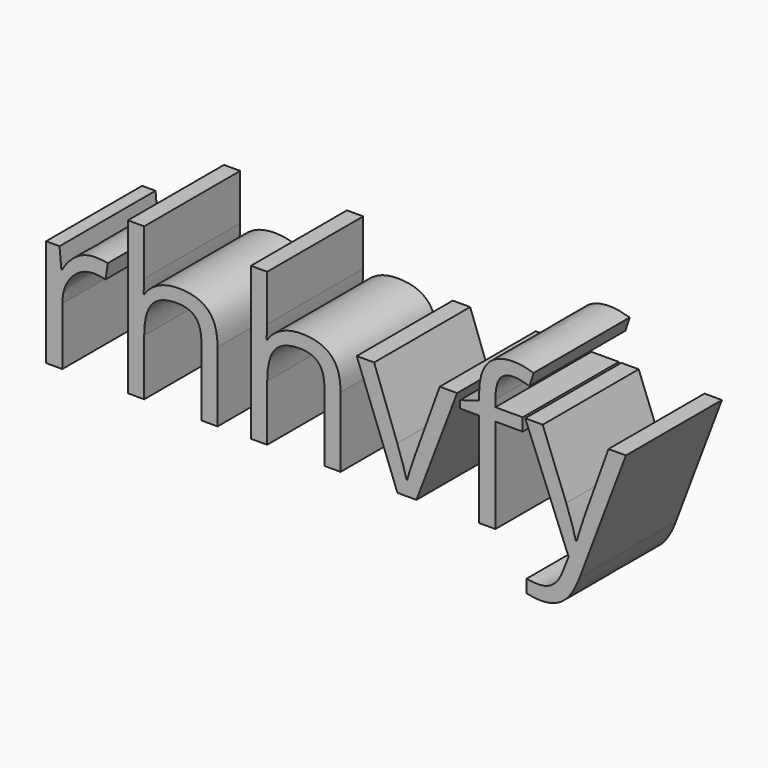
from build123d import *

# Parameters (mm, degrees)
F0_TEXT_SIZE = 42.4126784007
F1_DEPTH     = 25.4


# Not quite as in the source:
# - Text() gives the source's letters only with a copy of the font that has no kerning and outlines rounded to 1/6400 em; it was checked with that copy


with BuildPart() as f1:
    # F0 (on Front) → F1 (new body)
    with BuildSketch(Plane.XZ):
        with Locations((-47.7738343179, 49.2590814829)):
            Text('rhhvfy', F0_TEXT_SIZE, font='Open Sans', text_align=(TextAlign.LEFT, TextAlign.BOTTOM))
    extrude(amount=F1_DEPTH)


solid = f1.part
